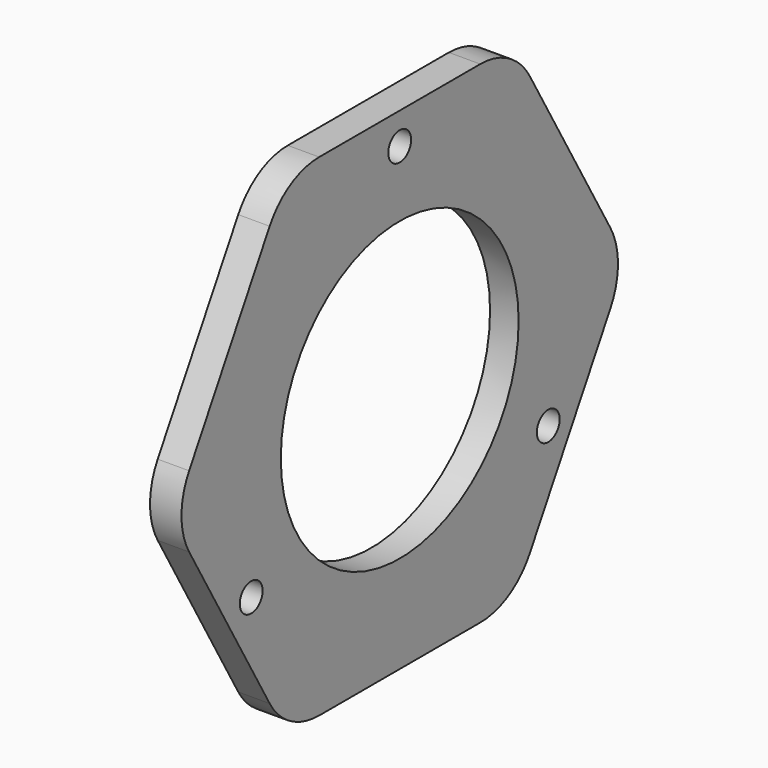
from build123d import *

# Parameters (mm, degrees)
F2_R             = 35.25
F3_DEPTH         = 11
F4_R             = 25
F7_R             = 17.5
F8_DEPTH         = 14.001
F9_R             = 5
F10_DEPTH        = 67.001
F10_COPIES_COUNT = 3
F11_R            = 52
F11_R_2          = 17.5
F12_DEPTH        = 67.001
F13_W            = 268.7109410763
F13_H            = 256.3393563032
F13_R            = 5
F13_R_2          = 52
F14_DEPTH        = 40
F15_R            = 63
F15_R_2          = 52
F16_DEPTH        = 1


# Not quite as in the source:
# - a feature of the source that left no trace in its solid (it failed there, or was rolled back) is left out
# - a pattern or mirror of a feature is missing from the dataset's text; its kind, count and spacing are read off the source's solid


with BuildPart() as f1:
    # F0 (on Front) → F1 (revolve)
    with BuildSketch(Plane.XZ):
        Polygon((67, 28.15), (67, 35.25), (0, 35.25), (0, 0), (14, 0), (14, 28.15), align=None)
    revolve(axis=Axis((7, 0, 0), (-1, 0, 0)))

    # F2 (on face) → F3 (join)
    with BuildSketch(Plane(origin=(0, 0, 0), x_dir=(0, -1, 0), z_dir=(-1, 0, 0))):
        Polygon((49.6521231503, 86), (-49.6521231503, 86), (-99.3042463006, 0), (-49.6521231503, -86), (49.6521231503, -86), (99.3042463006, 0), align=None)
        Circle(F2_R, mode=Mode.SUBTRACT)
    extrude(amount=-F3_DEPTH)

    # F4
    f4_edges = [f1.edges().sort_by_distance(p)[0] for p in [
        (5.5, 49.652123, -86),
        (5.5, -49.652123, -86),
        (5.5, -99.304246, 0),
        (5.5, -49.652123, 86),
        (5.5, 99.304246, 0),
        (5.5, 49.652123, 86),
    ]]
    fillet(f4_edges, radius=F4_R)

    # F7 (on face) → F8 (cut, through all)
    with BuildSketch(Plane.YZ.offset(14)):
        Circle(F7_R)
    extrude(amount=-F8_DEPTH, mode=Mode.SUBTRACT)

    # F9 (on face) → F10 (cut, through all)
    with BuildSketch(Plane(origin=(0, 0, 0), x_dir=(0, -1, 0), z_dir=(-1, 0, 0))):
        with Locations((-64.9519052838, -37.5)):
            Circle(F9_R)
    f10 = extrude(amount=-F10_DEPTH, mode=Mode.SUBTRACT)

    # F10_copies: F10 ×3 about axis
    f10_copies_axis = Axis((0, 0, 0), (1, 0, 0))
    for i in range(1, F10_COPIES_COUNT):
        add(f10.rotate(f10_copies_axis, i * 360 / F10_COPIES_COUNT), mode=Mode.SUBTRACT)

    # F11 (on face) → F12 (cut, through all)
    with BuildSketch(Plane(origin=(0, 0, 0), x_dir=(0, -1, 0), z_dir=(-1, 0, 0))):
        Circle(F11_R)
        Circle(F11_R_2, mode=Mode.SUBTRACT)
    extrude(amount=-F12_DEPTH, mode=Mode.SUBTRACT)

    # F13 (on face) → F14 (cut)
    with BuildSketch(Plane.YZ.offset(11)):
        with Locations((8.389338851, -8.3738937974)):
            Rectangle(F13_W, F13_H)
        with BuildLine():
            Line((-35.2183664206, 86), (35.2183664206, 86))
            ThreePointArc((35.2183664206, 86), (47.7183664206, 82.6506350946), (56.8690015152, 73.5))
            Line((56.8690015152, 73.5), (92.0873679357, 12.5))
            ThreePointArc((92.0873679357, 12.5), (95.4367328411, 0), (92.0873679357, -12.5))
            Line((92.0873679357, -12.5), (56.8690015152, -73.5))
            ThreePointArc((56.8690015152, -73.5), (47.7183664206, -82.6506350946), (35.2183664206, -86))
            Line((35.2183664206, -86), (-35.2183664206, -86))
            ThreePointArc((-35.2183664206, -86), (-47.7183664206, -82.6506350946), (-56.8690015152, -73.5))
            Line((-56.8690015152, -73.5), (-92.0873679357, -12.5))
            ThreePointArc((-92.0873679357, -12.5), (-95.4367328411, 0), (-92.0873679357, 12.5))
            Line((-92.0873679357, 12.5), (-56.8690015152, 73.5))
            ThreePointArc((-56.8690015152, 73.5), (-47.7183664206, 82.6506350946), (-35.2183664206, 86))
        make_face(mode=Mode.SUBTRACT)
        with BuildLine():
            ThreePointArc((56.8690015152, 73.5), (47.7183664206, 82.6506350946), (35.2183664206, 86))
            Line((35.2183664206, 86), (-35.2183664206, 86))
            ThreePointArc((-35.2183664206, 86), (-47.7183664206, 82.6506350946), (-56.8690015152, 73.5))
            Line((-56.8690015152, 73.5), (-92.0873679357, 12.5))
            ThreePointArc((-92.0873679357, 12.5), (-95.4367328411, 0), (-92.0873679357, -12.5))
            Line((-92.0873679357, -12.5), (-56.8690015152, -73.5))
            ThreePointArc((-56.8690015152, -73.5), (-47.7183664206, -82.6506350946), (-35.2183664206, -86))
            Line((-35.2183664206, -86), (35.2183664206, -86))
            ThreePointArc((35.2183664206, -86), (47.7183664206, -82.6506350946), (56.8690015152, -73.5))
            Line((56.8690015152, -73.5), (92.0873679357, -12.5))
            ThreePointArc((92.0873679357, -12.5), (95.4367328411, 0), (92.0873679357, 12.5))
            Line((92.0873679357, 12.5), (56.8690015152, 73.5))
        make_face()
        with Locations((-64.9519052838, -37.5)):
            Circle(F13_R, mode=Mode.SUBTRACT)
        with Locations((64.9519052838, -37.5)):
            Circle(F13_R, mode=Mode.SUBTRACT)
        Circle(F13_R_2, mode=Mode.SUBTRACT)
        with Locations((0, 75)):
            Circle(F13_R, mode=Mode.SUBTRACT)
    extrude(amount=F14_DEPTH, mode=Mode.SUBTRACT)

    # F15 (on face) → F16 (cut)
    with BuildSketch(Plane(origin=(0, 0, 0), x_dir=(0, -1, 0), z_dir=(-1, 0, 0))):
        Circle(F15_R)
        Circle(F15_R_2, mode=Mode.SUBTRACT)
    extrude(amount=-F16_DEPTH, mode=Mode.SUBTRACT)


solid = f1.part
